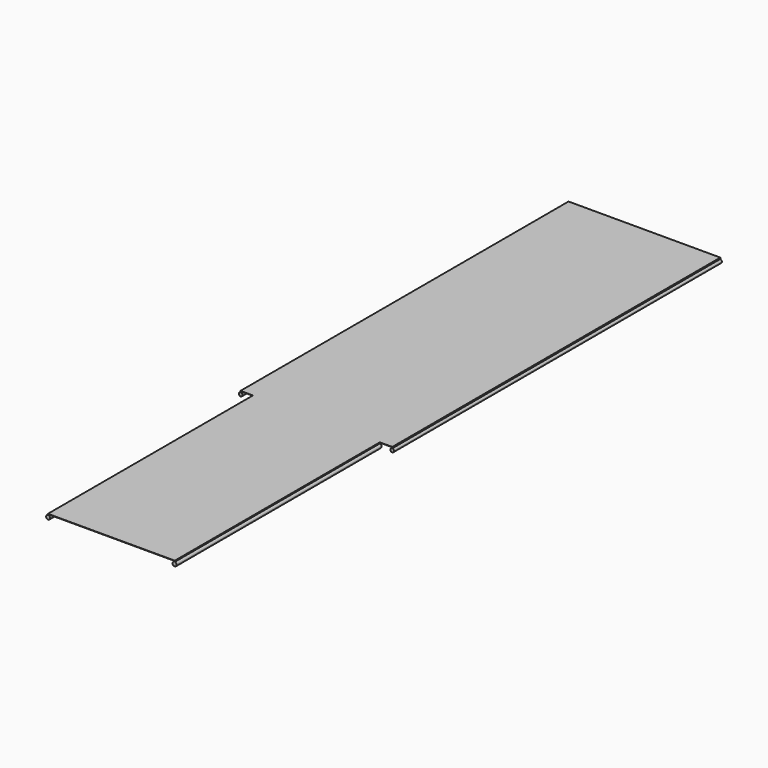
from build123d import *

# Parameters (mm, degrees)
F2_DEPTH  = 1910
F7_DEPTH  = 1120
F9_DEPTH  = 2000
F11_DEPTH = 700


# Not quite as in the source:
# - ends of sketch curves that miss each other by under 0.0002 mm in the source are joined


with BuildPart() as f2:
    # F1 (on Front) → F2 (new body)
    with BuildSketch(Plane.XZ):
        with BuildLine():
            Line((7.5, 37.974085065), (7.5, 40))
            Line((7.5, 40), (-15, 40))
            Line((-15, 40), (-15, 37))
            Line((-15, 37), (-15, 31))
            Line((-15, 31), (-15, 29))
            Line((-15, 29), (-15, 26))
            Line((-15, 26), (-15, 24))
            Line((-15, 24), (-13, 24))
            Line((-13, 24), (-11, 24))
            Line((-11, 24), (-11, 26))
            Line((-11, 26), (-9, 26))
            Line((-9, 26), (-9, 20))
            Line((-9, 20), (-11, 20))
            Line((-11, 20), (-11, 22))
            Line((-11, 22), (-15, 22))
            Line((-15, 22), (-15, 18))
            Line((-15, 18), (-15, 7.7))
            Line((-15, 7.7), (-13, 7.7))
            Line((-13, 7.7), (-13, 11.4920835048))
            Line((-13, 11.4920835048), (-7, 11.4920835048))
            Line((-7, 11.4920835048), (-7, 3.7))
            Line((-7, 3.7), (-11, 3.7))
            Line((-11, 3.7), (-11, 5.7))
            Line((-11, 5.7), (-15, 5.7))
            Line((-15, 5.7), (-15, 3))
            Line((-15, 3), (-15, 0))
            Line((-15, 0), (-13, 0))
            Line((-13, 0), (-12, 0))
            Line((-12, 0), (-5, 0))
            Line((-5, 0), (-5, 13.4920835048))
            Line((-5, 13.4920835048), (-7, 13.4920835048))
            Line((-7, 13.4920835048), (-9.1588944197, 13.4920835048))
            Line((-9.1588944197, 13.4920835048), (-9.1588944197, 15.4920835048))
            Line((-9.1588944197, 15.4920835048), (1.5, 20))
            Line((1.5, 20), (10.8411055803, 15.4920835048))
            Line((10.8411055803, 15.4920835048), (10.8411055803, 13.4920835048))
            Line((10.8411055803, 13.4920835048), (8, 13.4920835048))
            Line((8, 13.4920835048), (8, 0))
            Line((8, 0), (17, 0))
            Line((17, 0), (17, 40))
            Line((17, 40), (8.5, 40))
            Line((8.5, 40), (8.5, 37.974085065))
            ThreePointArc((8.5, 37.974085065), (11.5604089792, 36.6859489396), (13.3185590744, 33.8691589154))
            Line((13.3185590744, 33.8691589154), (13.4318527537, 31.7073867348))
            ThreePointArc((13.4318527537, 31.7073867348), (4.0126863822, 28.7323088758), (7.5, 37.974085065))
        make_face()
        Polygon((-8.3634709733, 18), (-11.1588944197, 16.817744602), (-11.1588944197, 15.4920835048), (-11.1588944197, 13.4920835048), (-13, 13.4920835048), (-13, 18), align=None, mode=Mode.SUBTRACT)
        with BuildLine():
            Line((-13, 34), (-13, 37.9999987781))
            Line((-13, 37.9999987781), (2.9081163149, 37.9999987781))
            ThreePointArc((2.9081163149, 37.9999987781), (3.810445381, 26.2974906682), (15, 29.8410427327))
            Line((15, 29.8410427327), (15, 2))
            Line((15, 2), (10, 2))
            Line((10, 2), (10, 12))
            Line((10, 12), (12.8411055803, 12))
            Line((12.8411055803, 12), (12.8411055803, 16.7476188273))
            Line((12.8411055803, 16.7476188273), (1.5543358685, 22.194491783))
            Line((1.5543358685, 22.194491783), (-7, 18.5766464184))
            Line((-7, 18.5766464184), (-7, 28))
            Line((-7, 28), (-13, 28))
            Line((-13, 28), (-13, 34))
        make_face(mode=Mode.SUBTRACT)
        with BuildLine():
            Line((13.0918836851, 37.9999987781), (13.1020709306, 37.9999987781))
            Line((13.1020709306, 37.9999987781), (13.1025921338, 37.9900536295))
            ThreePointArc((13.1025921338, 37.9900536295), (13.0972403349, 37.9950288154), (13.0918836851, 37.9999987781))
        make_face(mode=Mode.SUBTRACT)
    extrude(amount=-F2_DEPTH)

    # F6 (on Front) → F7 (join)
    with BuildSketch(Plane.XZ):
        with BuildLine():
            Line((8.5, 37.3712719703), (8.5, 40))
            Line((8.5, 40), (8.5, 41))
            Line((8.5, 41), (-198.8, 41))
            Line((-198.8, 41), (-198.8, 40))
            Line((-198.8, 40), (-25.5, 40))
            Line((-25.5, 40), (-15, 40))
            Line((-15, 40), (7.5, 40))
            Line((7.5, 40), (7.5, 37.3712723193))
            ThreePointArc((7.5, 37.3712723193), (7.9999999822, 27.6162403216), (8.5, 37.3712719703))
        make_face()
    extrude(amount=-F7_DEPTH)

    # F8 (on face) → F9 (cut)
    with BuildSketch(Plane.XZ):
        with BuildLine():
            Line((-15, 3), (-15, 0))
            Line((-15, 0), (-13, 0))
            Line((-13, 0), (-12, 0))
            Line((-12, 0), (-5, 0))
            Line((-5, 0), (-5, 13.4920835048))
            Line((-5, 13.4920835048), (-7, 13.4920835048))
            Line((-7, 13.4920835048), (-9.1588944197, 13.4920835048))
            Line((-9.1588944197, 13.4920835048), (-9.1588944197, 15.4920835048))
            Line((-9.1588944197, 15.4920835048), (1.5, 20))
            Line((1.5, 20), (10.8411055803, 15.4920835048))
            Line((10.8411055803, 15.4920835048), (10.8411055803, 13.4920835048))
            Line((10.8411055803, 13.4920835048), (8, 13.4920835048))
            Line((8, 13.4920835048), (8, 0))
            Line((8, 0), (17, 0))
            Line((17, 0), (17, 40))
            Line((17, 40), (8.5, 40))
            Line((8.5, 40), (8.5, 37.974085065))
            ThreePointArc((8.5, 37.974085065), (11.5604089792, 36.6859489396), (13.3185590744, 33.8691589154))
            Line((13.3185590744, 33.8691589154), (13.4318527537, 31.7073867348))
            ThreePointArc((13.4318527537, 31.7073867348), (4.0126863822, 28.7323088758), (7.5, 37.974085065))
            Line((7.5, 37.974085065), (7.5, 40))
            Line((7.5, 40), (-15, 40))
            Line((-15, 40), (-15, 31))
            Line((-15, 31), (-15, 29))
            Line((-15, 29), (-15, 24))
            Line((-15, 24), (-13, 24))
            Line((-13, 24), (-11, 24))
            Line((-11, 24), (-11, 26))
            Line((-11, 26), (-9, 26))
            Line((-9, 26), (-9, 20))
            Line((-9, 20), (-11, 20))
            Line((-11, 20), (-11, 22))
            Line((-11, 22), (-15, 22))
            Line((-15, 22), (-15, 18))
            Line((-15, 18), (-15, 7.7))
            Line((-15, 7.7), (-13, 7.7))
            Line((-13, 7.7), (-13, 11.4920835048))
            Line((-13, 11.4920835048), (-7, 11.4920835048))
            Line((-7, 11.4920835048), (-7, 3.7))
            Line((-7, 3.7), (-11, 3.7))
            Line((-11, 3.7), (-11, 5.7))
            Line((-11, 5.7), (-15, 5.7))
            Line((-15, 5.7), (-15, 3))
        make_face()
        Polygon((-13, 18), (-8.3634709733, 18), (-11.1588944197, 16.817744602), (-11.1588944197, 15.4920835048), (-11.1588944197, 13.4920835048), (-13, 13.4920835048), align=None, mode=Mode.SUBTRACT)
        with BuildLine():
            Line((12.8411055803, 12), (12.8411055803, 16.7476188273))
            Line((12.8411055803, 16.7476188273), (1.5543358685, 22.194491783))
            Line((1.5543358685, 22.194491783), (-7, 18.5766464184))
            Line((-7, 18.5766464184), (-7, 28))
            Line((-7, 28), (-13, 28))
            Line((-13, 28), (-13, 34))
            Line((-13, 34), (-13, 37.9999987781))
            Line((-13, 37.9999987781), (2.9081163149, 37.9999987781))
            ThreePointArc((2.9081163149, 37.9999987781), (3.810445381, 26.2974906682), (15, 29.8410427327))
            Line((15, 29.8410427327), (15, 2))
            Line((15, 2), (10, 2))
            Line((10, 2), (10, 12))
            Line((10, 12), (12.8411055803, 12))
        make_face(mode=Mode.SUBTRACT)
    extrude(amount=-F9_DEPTH, mode=Mode.SUBTRACT)

    # F10 (on face) → F11 (join)
    with BuildSketch(Plane.XZ):
        with BuildLine():
            Line((-49.096, 40), (-26.596, 40))
            Line((-26.596, 40), (-26.596, 37.9675733099))
            ThreePointArc((-26.596, 37.9675733099), (-25.951759356, 27.0133522571), (-25.5, 37.9771982231))
            Line((-25.5, 37.9771982231), (-25.5, 41))
            Line((-25.5, 41), (-198.8, 41))
            Line((-198.8, 41), (-198.8, 40))
            Line((-198.8, 40), (-49.096, 40))
        make_face()
    extrude(amount=F11_DEPTH)

    # F12: F2 across face


with BuildPart() as f2_1:
    add(f2.part)
    add(f2.part.mirror(Plane(origin=(-198.8, 210, 40.5), x_dir=(0, -1, 0), z_dir=(-1, 0, 0))))


solid = f2_1.part
